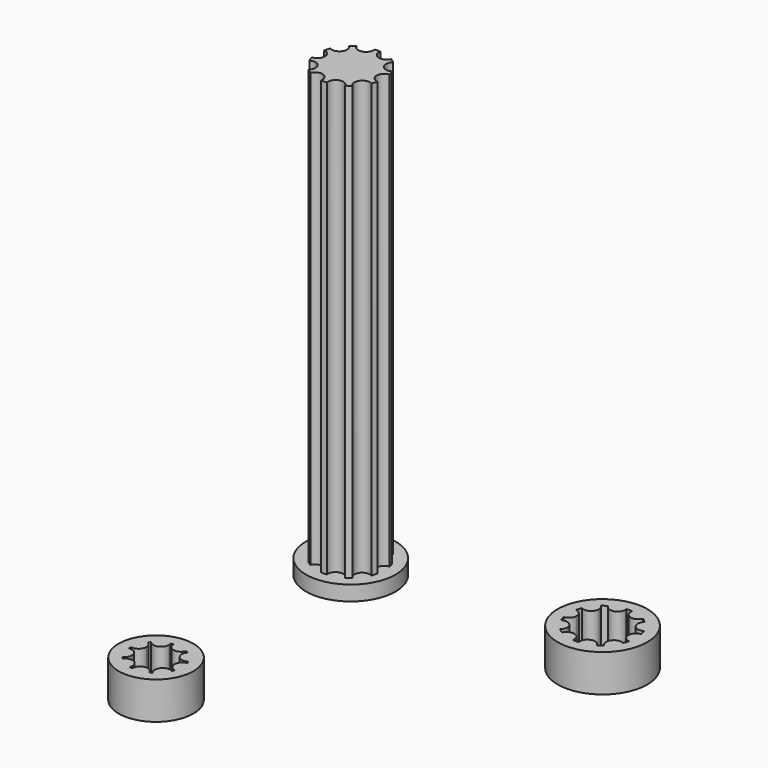
from build123d import *

# Parameters (mm, degrees)
F0_R            = 4.5
F1_DEPTH        = 60
F0_R_2          = 6
F2_DEPTH        = 2
F3_R            = 1.0345297628
F4_DEPTH        = 58
F4_COPIES_COUNT = 10
F6_R            = 1.3
F7_DEPTH        = 25
F8_R            = 6
F9_DEPTH        = 5
F10_R           = 5
F11_DEPTH       = 5


# Not quite as in the source:
# - a pattern or mirror of a feature is missing from the dataset's text; its kind, count and spacing are read off the source's solid


with BuildPart() as f1:
    # F0 (on Top) → F1 (new body)
    with BuildSketch(Plane.XY):
        Circle(F0_R)
    extrude(amount=F1_DEPTH)

    # F0 (on Top) → F2 (join)
    with BuildSketch(Plane.XY):
        Circle(F0_R_2)
        Circle(F0_R, mode=Mode.SUBTRACT)
    extrude(amount=F2_DEPTH)

    # F3 (on face) → F4 (cut)
    with BuildSketch(Plane.XY.offset(60)):
        with Locations((4.5, 0)):
            Circle(F3_R)
    f4 = extrude(amount=-F4_DEPTH, mode=Mode.SUBTRACT)

    # F4_copies: F4 ×10 about axis
    f4_copies_axis = Axis((0, 0, 0), (0, 0, 1))
    for i in range(1, F4_COPIES_COUNT):
        add(f4.rotate(f4_copies_axis, i * 360 / F4_COPIES_COUNT), mode=Mode.SUBTRACT)

    # F6 (on face) → F7 (cut)
    with BuildSketch(Plane.XY):
        Circle(F6_R)
    extrude(amount=F7_DEPTH, mode=Mode.SUBTRACT)


with BuildPart() as f9:
    # F8 (on Top) → F9 (new body)
    with BuildSketch(Plane.XY):
        with Locations((33.7035082627, 0)):
            Circle(F8_R)
        with BuildLine():
            ThreePointArc((37.8519180528, 1.7437592189), (37.983262586, 1.3905764747), (38.0845982349, 1.0276432529))
            ThreePointArc((38.0845982349, 1.0276432529), (38.8916862289, 0.7723997261), (39.2380082627, 0))
            ThreePointArc((39.2380082627, 0), (38.8916862289, -0.7723997261), (38.0845982349, -1.0276432529))
            ThreePointArc((38.0845982349, -1.0276432529), (37.983262586, -1.3905764747), (37.8519180528, -1.7437592189))
            ThreePointArc((37.8519180528, -1.7437592189), (38.2372655183, -2.1230965293), (38.3785847374, -2.6450336353))
            ThreePointArc((38.3785847374, -2.6450336353), (37.7598962347, -3.5922881147), (36.6438509554, -3.4065209304))
            ThreePointArc((36.6438509554, -3.4065209304), (36.348541898, -3.6405764747), (36.0346863301, -3.8491049372))
            ThreePointArc((36.0346863301, -3.8491049372), (36.1048375751, -4.0593706779), (36.1285847374, -4.2797543233))
            ThreePointArc((36.1285847374, -4.2797543233), (35.1968272393, -5.3091396877), (34.0799927059, -4.4842233959))
            ThreePointArc((34.0799927059, -4.4842233959), (33.7035082627, -4.5), (33.3270238195, -4.4842233959))
            ThreePointArc((33.3270238195, -4.4842233959), (31.9932537074, -5.2636222894), (31.3723301953, -3.8491049372))
            ThreePointArc((31.3723301953, -3.8491049372), (31.0584746274, -3.6405764747), (30.76316557, -3.4065209304))
            ThreePointArc((30.76316557, -3.4065209304), (29.2260037074, -3.2530974788), (29.5550984726, -1.7437592189))
            ThreePointArc((29.5550984726, -1.7437592189), (29.4237539394, -1.3905764747), (29.3224182905, -1.0276432529))
            ThreePointArc((29.3224182905, -1.0276432529), (28.1690082627, 0), (29.3224182905, 1.0276432529))
            ThreePointArc((29.3224182905, 1.0276432529), (29.4237539394, 1.3905764747), (29.5550984726, 1.7437592189))
            ThreePointArc((29.5550984726, 1.7437592189), (29.2260037074, 3.2530974788), (30.76316557, 3.4065209304))
            ThreePointArc((30.76316557, 3.4065209304), (31.0584746274, 3.6405764747), (31.3723301953, 3.8491049372))
            ThreePointArc((31.3723301953, 3.8491049372), (31.9932537074, 5.2636222894), (33.3270238195, 4.4842233959))
            ThreePointArc((33.3270238195, 4.4842233959), (33.7035082627, 4.5), (34.0799927059, 4.4842233959))
            ThreePointArc((34.0799927059, 4.4842233959), (35.1968272393, 5.3091396877), (36.1285847374, 4.2797543233))
            ThreePointArc((36.1285847374, 4.2797543233), (36.1048375751, 4.0593706779), (36.0346863301, 3.8491049372))
            ThreePointArc((36.0346863301, 3.8491049372), (36.348541898, 3.6405764747), (36.6438509554, 3.4065209304))
            ThreePointArc((36.6438509554, 3.4065209304), (37.7598962347, 3.5922881147), (38.3785847374, 2.6450336353))
            ThreePointArc((38.3785847374, 2.6450336353), (38.2372655183, 2.1230965293), (37.8519180528, 1.7437592189))
        make_face(mode=Mode.SUBTRACT)
        with BuildLine():
            ThreePointArc((38.3785847374, -2.6450336353), (38.2372655183, -2.1230965293), (37.8519180528, -1.7437592189))
            ThreePointArc((37.8519180528, -1.7437592189), (37.3440847374, -2.6450336353), (36.6438509554, -3.4065209304))
            ThreePointArc((36.6438509554, -3.4065209304), (37.7598962347, -3.5922881147), (38.3785847374, -2.6450336353))
        make_face()
        with BuildLine():
            ThreePointArc((36.1285847374, -4.2797543233), (36.1048375751, -4.0593706779), (36.0346863301, -3.8491049372))
            ThreePointArc((36.0346863301, -3.8491049372), (35.0940847374, -4.2797543233), (34.0799927059, -4.4842233959))
            ThreePointArc((34.0799927059, -4.4842233959), (35.1968272393, -5.3091396877), (36.1285847374, -4.2797543233))
        make_face()
        with BuildLine():
            ThreePointArc((31.3723301953, -3.8491049372), (31.9932537074, -5.2636222894), (33.3270238195, -4.4842233959))
            ThreePointArc((33.3270238195, -4.4842233959), (32.312931788, -4.2797543233), (31.3723301953, -3.8491049372))
        make_face()
        with BuildLine():
            ThreePointArc((29.5550984726, -1.7437592189), (29.2260037074, -3.2530974788), (30.76316557, -3.4065209304))
            ThreePointArc((30.76316557, -3.4065209304), (30.062931788, -2.6450336353), (29.5550984726, -1.7437592189))
        make_face()
        with BuildLine():
            ThreePointArc((29.3224182905, -1.0276432529), (29.2035082627, 0), (29.3224182905, 1.0276432529))
            ThreePointArc((29.3224182905, 1.0276432529), (28.1690082627, 0), (29.3224182905, -1.0276432529))
        make_face()
        with BuildLine():
            ThreePointArc((29.5550984726, 1.7437592189), (30.062931788, 2.6450336353), (30.76316557, 3.4065209304))
            ThreePointArc((30.76316557, 3.4065209304), (29.2260037074, 3.2530974788), (29.5550984726, 1.7437592189))
        make_face()
        with BuildLine():
            ThreePointArc((31.3723301953, 3.8491049372), (32.312931788, 4.2797543233), (33.3270238195, 4.4842233959))
            ThreePointArc((33.3270238195, 4.4842233959), (31.9932537074, 5.2636222894), (31.3723301953, 3.8491049372))
        make_face()
        with BuildLine():
            ThreePointArc((34.0799927059, 4.4842233959), (35.0940847374, 4.2797543233), (36.0346863301, 3.8491049372))
            ThreePointArc((36.0346863301, 3.8491049372), (36.1048375751, 4.0593706779), (36.1285847374, 4.2797543233))
            ThreePointArc((36.1285847374, 4.2797543233), (35.1968272393, 5.3091396877), (34.0799927059, 4.4842233959))
        make_face()
        with BuildLine():
            ThreePointArc((36.6438509554, 3.4065209304), (37.3440847374, 2.6450336353), (37.8519180528, 1.7437592189))
            ThreePointArc((37.8519180528, 1.7437592189), (38.2372655183, 2.1230965293), (38.3785847374, 2.6450336353))
            ThreePointArc((38.3785847374, 2.6450336353), (37.7598962347, 3.5922881147), (36.6438509554, 3.4065209304))
        make_face()
        with BuildLine():
            ThreePointArc((38.0845982349, 1.0276432529), (38.1736819101, 0.51725), (38.2035082627, 0))
            ThreePointArc((38.2035082627, 0), (38.1736819101, -0.51725), (38.0845982349, -1.0276432529))
            ThreePointArc((38.0845982349, -1.0276432529), (38.8916862289, -0.7723997261), (39.2380082627, 0))
            ThreePointArc((39.2380082627, 0), (38.8916862289, 0.7723997261), (38.0845982349, 1.0276432529))
        make_face()
        with BuildLine():
            ThreePointArc((34.0799927059, -4.4842233959), (35.0940847374, -4.2797543233), (36.0346863301, -3.8491049372))
            ThreePointArc((36.0346863301, -3.8491049372), (34.7744066567, -3.2958863572), (34.0799927059, -4.4842233959))
        make_face()
        with BuildLine():
            ThreePointArc((31.3723301953, -3.8491049372), (32.312931788, -4.2797543233), (33.3270238195, -4.4842233959))
            ThreePointArc((33.3270238195, -4.4842233959), (33.3423171524, -4.3824968252), (33.347431788, -4.2797543233))
            ThreePointArc((33.347431788, -4.2797543233), (32.5333154334, -3.2690014857), (31.3723301953, -3.8491049372))
        make_face()
        with BuildLine():
            ThreePointArc((29.5550984726, -1.7437592189), (30.062931788, -2.6450336353), (30.76316557, -3.4065209304))
            ThreePointArc((30.76316557, -3.4065209304), (31.0101862674, -3.0608451326), (31.097431788, -2.6450336353))
            ThreePointArc((31.097431788, -2.6450336353), (30.584868894, -1.7518528544), (29.5550984726, -1.7437592189))
        make_face()
        with BuildLine():
            ThreePointArc((36.6438509554, -3.4065209304), (37.3440847374, -2.6450336353), (37.8519180528, -1.7437592189))
            ThreePointArc((37.8519180528, -1.7437592189), (36.5071566567, -2.0369697918), (36.6438509554, -3.4065209304))
        make_face()
        with BuildLine():
            ThreePointArc((30.2380082627, 0), (29.9759079888, 0.6881779662), (29.3224182905, 1.0276432529))
            ThreePointArc((29.3224182905, 1.0276432529), (29.2035082627, 0), (29.3224182905, -1.0276432529))
            ThreePointArc((29.3224182905, -1.0276432529), (29.9759079888, -0.6881779662), (30.2380082627, 0))
        make_face()
        with BuildLine():
            ThreePointArc((31.097431788, 2.6450336353), (31.0101862674, 3.0608451326), (30.76316557, 3.4065209304))
            ThreePointArc((30.76316557, 3.4065209304), (30.062931788, 2.6450336353), (29.5550984726, 1.7437592189))
            ThreePointArc((29.5550984726, 1.7437592189), (30.584868894, 1.7518528544), (31.097431788, 2.6450336353))
        make_face()
        with BuildLine():
            ThreePointArc((33.347431788, 4.2797543233), (33.3423171524, 4.3824968252), (33.3270238195, 4.4842233959))
            ThreePointArc((33.3270238195, 4.4842233959), (32.312931788, 4.2797543233), (31.3723301953, 3.8491049372))
            ThreePointArc((31.3723301953, 3.8491049372), (32.5333154334, 3.2690014857), (33.347431788, 4.2797543233))
        make_face()
        with BuildLine():
            ThreePointArc((34.0799927059, 4.4842233959), (34.7744066567, 3.2958863572), (36.0346863301, 3.8491049372))
            ThreePointArc((36.0346863301, 3.8491049372), (35.0940847374, 4.2797543233), (34.0799927059, 4.4842233959))
        make_face()
        with BuildLine():
            ThreePointArc((36.6438509554, 3.4065209304), (36.5071566567, 2.0369697918), (37.8519180528, 1.7437592189))
            ThreePointArc((37.8519180528, 1.7437592189), (37.3440847374, 2.6450336353), (36.6438509554, 3.4065209304))
        make_face()
        with BuildLine():
            ThreePointArc((38.0845982349, -1.0276432529), (38.1736819101, -0.51725), (38.2035082627, 0))
            ThreePointArc((38.2035082627, 0), (38.1736819101, 0.51725), (38.0845982349, 1.0276432529))
            ThreePointArc((38.0845982349, 1.0276432529), (37.1690082627, 0), (38.0845982349, -1.0276432529))
        make_face()
    extrude(amount=F9_DEPTH)


with BuildPart() as f11:
    # F10 (on Top) → F11 (new body)
    with BuildSketch(Plane.XY):
        with Locations((1.7561594723, -34.7853899002)):
            Circle(F10_R)
        with BuildLine():
            ThreePointArc((4.9778609223, -33.4176765651), (5.045083645, -33.5883193986), (5.1032751509, -33.7622493262))
            ThreePointArc((5.1032751509, -33.7622493262), (5.9314488249, -34.0016970138), (6.2906594723, -34.7853899002))
            ThreePointArc((6.2906594723, -34.7853899002), (5.9314488249, -35.5690827866), (5.1032751509, -35.8085304743))
            ThreePointArc((5.1032751509, -35.8085304743), (5.045083645, -35.9824604018), (4.9778609223, -36.1531032353))
            ThreePointArc((4.9778609223, -36.1531032353), (5.3399181981, -36.5296786729), (5.4718150232, -37.0351465341))
            ThreePointArc((5.4718150232, -37.0351465341), (4.8038406914, -38.0025395176), (3.6625367544, -37.7206455379))
            ThreePointArc((3.6625367544, -37.7206455379), (3.5061594723, -37.8164788135), (3.34497678, -37.9039888745))
            ThreePointArc((3.34497678, -37.9039888745), (3.3849778274, -38.0659410838), (3.3984280941, -38.2322170358))
            ThreePointArc((3.3984280941, -38.2322170358), (2.377481673, -39.2666282453), (1.3297832406, -38.2593218669))
            ThreePointArc((1.3297832406, -38.2593218669), (1.1483908504, -38.2322170358), (0.9686673618, -38.1956473943))
            ThreePointArc((0.9686673618, -38.1956473943), (-0.5110905277, -38.7123820937), (-0.8034640958, -37.1725068202))
            ThreePointArc((-0.8034640958, -37.1725068202), (-0.9249960786, -37.0351465341), (-1.039165746, -36.8916085318))
            ThreePointArc((-1.039165746, -36.8916085318), (-2.5048767167, -36.3362802401), (-1.7390351176, -34.9687332369))
            ThreePointArc((-1.7390351176, -34.9687332369), (-1.7438405277, -34.7853899002), (-1.7390351176, -34.6020465636))
            ThreePointArc((-1.7390351176, -34.6020465636), (-2.5048767167, -33.2344995603), (-1.039165746, -32.6791712686))
            ThreePointArc((-1.039165746, -32.6791712686), (-0.9249960786, -32.5356332663), (-0.8034640958, -32.3982729802))
            ThreePointArc((-0.8034640958, -32.3982729802), (-0.5110905277, -30.8583977067), (0.9686673618, -31.3751324061))
            ThreePointArc((0.9686673618, -31.3751324061), (1.1483908504, -31.3385627647), (1.3297832406, -31.3114579335))
            ThreePointArc((1.3297832406, -31.3114579335), (2.377481673, -30.3041515551), (3.3984280941, -31.3385627647))
            ThreePointArc((3.3984280941, -31.3385627647), (3.3849778274, -31.5048387166), (3.34497678, -31.6667909259))
            ThreePointArc((3.34497678, -31.6667909259), (3.5061594723, -31.754300987), (3.6625367544, -31.8501342626))
            ThreePointArc((3.6625367544, -31.8501342626), (4.8038406914, -31.5682402828), (5.4718150232, -32.5356332663))
            ThreePointArc((5.4718150232, -32.5356332663), (5.3399181981, -33.0411011275), (4.9778609223, -33.4176765651))
        make_face(mode=Mode.SUBTRACT)
        with BuildLine():
            ThreePointArc((1.3297832406, -31.3114579335), (2.3639280941, -31.3385627647), (3.34497678, -31.6667909259))
            ThreePointArc((3.34497678, -31.6667909259), (3.3849778274, -31.5048387166), (3.3984280941, -31.3385627647))
            ThreePointArc((3.3984280941, -31.3385627647), (2.377481673, -30.3041515551), (1.3297832406, -31.3114579335))
        make_face()
        with BuildLine():
            ThreePointArc((3.6625367544, -31.8501342626), (4.4373150232, -32.5356332663), (4.9778609223, -33.4176765651))
            ThreePointArc((4.9778609223, -33.4176765651), (5.3399181981, -33.0411011275), (5.4718150232, -32.5356332663))
            ThreePointArc((5.4718150232, -32.5356332663), (4.8038406914, -31.5682402828), (3.6625367544, -31.8501342626))
        make_face()
        with BuildLine():
            ThreePointArc((5.1032751509, -33.7622493262), (5.2177273883, -34.2681399002), (5.2561594723, -34.7853899002))
            ThreePointArc((5.2561594723, -34.7853899002), (5.2177273883, -35.3026399002), (5.1032751509, -35.8085304743))
            ThreePointArc((5.1032751509, -35.8085304743), (5.9314488249, -35.5690827866), (6.2906594723, -34.7853899002))
            ThreePointArc((6.2906594723, -34.7853899002), (5.9314488249, -34.0016970138), (5.1032751509, -33.7622493262))
        make_face()
        with BuildLine():
            ThreePointArc((5.4718150232, -37.0351465341), (5.3399181981, -36.5296786729), (4.9778609223, -36.1531032353))
            ThreePointArc((4.9778609223, -36.1531032353), (4.4373150232, -37.0351465341), (3.6625367544, -37.7206455379))
            ThreePointArc((3.6625367544, -37.7206455379), (4.8038406914, -38.0025395176), (5.4718150232, -37.0351465341))
        make_face()
        with BuildLine():
            ThreePointArc((3.3984280941, -38.2322170358), (3.3849778274, -38.0659410838), (3.34497678, -37.9039888745))
            ThreePointArc((3.34497678, -37.9039888745), (2.3639280941, -38.2322170358), (1.3297832406, -38.2593218669))
            ThreePointArc((1.3297832406, -38.2593218669), (2.377481673, -39.2666282453), (3.3984280941, -38.2322170358))
        make_face()
        with BuildLine():
            ThreePointArc((-0.8034640958, -37.1725068202), (-0.5110905277, -38.7123820937), (0.9686673618, -38.1956473943))
            ThreePointArc((0.9686673618, -38.1956473943), (0.0061594723, -37.8164788135), (-0.8034640958, -37.1725068202))
        make_face()
        with BuildLine():
            ThreePointArc((-1.7390351176, -34.9687332369), (-2.5048767167, -36.3362802401), (-1.039165746, -36.8916085318))
            ThreePointArc((-1.039165746, -36.8916085318), (-1.5327647005, -35.9824604018), (-1.7390351176, -34.9687332369))
        make_face()
        with BuildLine():
            ThreePointArc((-1.7390351176, -34.6020465636), (-1.5327647005, -33.5883193986), (-1.039165746, -32.6791712686))
            ThreePointArc((-1.039165746, -32.6791712686), (-2.5048767167, -33.2344995603), (-1.7390351176, -34.6020465636))
        make_face()
        with BuildLine():
            ThreePointArc((-0.8034640958, -32.3982729802), (0.0061594723, -31.754300987), (0.9686673618, -31.3751324061))
            ThreePointArc((0.9686673618, -31.3751324061), (-0.5110905277, -30.8583977067), (-0.8034640958, -32.3982729802))
        make_face()
        with BuildLine():
            ThreePointArc((1.3297832406, -31.3114579335), (2.1842890543, -32.3573463852), (3.34497678, -31.6667909259))
            ThreePointArc((3.34497678, -31.6667909259), (2.3639280941, -31.3385627647), (1.3297832406, -31.3114579335))
        make_face()
        with BuildLine():
            ThreePointArc((3.6625367544, -31.8501342626), (3.6448420468, -33.2005970485), (4.9778609223, -33.4176765651))
            ThreePointArc((4.9778609223, -33.4176765651), (4.4373150232, -32.5356332663), (3.6625367544, -31.8501342626))
        make_face()
        with BuildLine():
            ThreePointArc((5.1032751509, -35.8085304743), (5.2177273883, -35.3026399002), (5.2561594723, -34.7853899002))
            ThreePointArc((5.2561594723, -34.7853899002), (5.2177273883, -34.2681399002), (5.1032751509, -33.7622493262))
            ThreePointArc((5.1032751509, -33.7622493262), (4.2216594723, -34.7853899002), (5.1032751509, -35.8085304743))
        make_face()
        with BuildLine():
            ThreePointArc((1.3297832406, -38.2593218669), (2.3639280941, -38.2322170358), (3.34497678, -37.9039888745))
            ThreePointArc((3.34497678, -37.9039888745), (2.1842890543, -37.2134334153), (1.3297832406, -38.2593218669))
        make_face()
        with BuildLine():
            ThreePointArc((-0.8034640958, -37.1725068202), (0.0061594723, -37.8164788135), (0.9686673618, -38.1956473943))
            ThreePointArc((0.9686673618, -38.1956473943), (1.022502097, -38.0094501045), (1.0406594723, -37.8164788135))
            ThreePointArc((1.0406594723, -37.8164788135), (0.3472127444, -36.839814636), (-0.8034640958, -37.1725068202))
        make_face()
        with BuildLine():
            ThreePointArc((-1.7390351176, -34.9687332369), (-1.5327647005, -35.9824604018), (-1.039165746, -36.8916085318))
            ThreePointArc((-1.039165746, -36.8916085318), (-0.6437151044, -36.5114037502), (-0.4982647005, -35.9824604018))
            ThreePointArc((-0.4982647005, -35.9824604018), (-0.8782406354, -35.1813433703), (-1.7390351176, -34.9687332369))
        make_face()
        with BuildLine():
            ThreePointArc((-0.4982647005, -33.5883193986), (-0.6437151044, -33.0593760502), (-1.039165746, -32.6791712686))
            ThreePointArc((-1.039165746, -32.6791712686), (-1.5327647005, -33.5883193986), (-1.7390351176, -34.6020465636))
            ThreePointArc((-1.7390351176, -34.6020465636), (-0.8782406354, -34.3894364301), (-0.4982647005, -33.5883193986))
        make_face()
        with BuildLine():
            ThreePointArc((1.0406594723, -31.754300987), (1.022502097, -31.5613296959), (0.9686673618, -31.3751324061))
            ThreePointArc((0.9686673618, -31.3751324061), (0.0061594723, -31.754300987), (-0.8034640958, -32.3982729802))
            ThreePointArc((-0.8034640958, -32.3982729802), (0.3472127444, -32.7309651644), (1.0406594723, -31.754300987))
        make_face()
        with BuildLine():
            ThreePointArc((3.6625367544, -37.7206455379), (4.4373150232, -37.0351465341), (4.9778609223, -36.1531032353))
            ThreePointArc((4.9778609223, -36.1531032353), (3.6448420468, -36.3701827519), (3.6625367544, -37.7206455379))
        make_face()
    extrude(amount=F11_DEPTH)


solid = Compound([f1.part, f9.part, f11.part])
